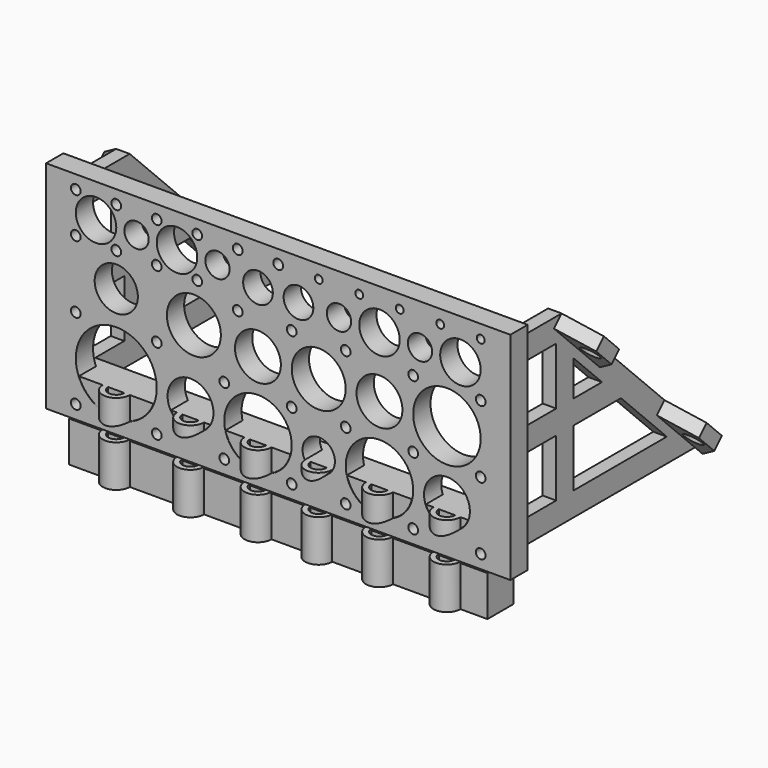
from build123d import *

# Parameters (mm, degrees)
F0_R            = 1.8
F0_R_2          = 1.45
F1_DEPTH        = 8
F2_R            = 8.5
F2_R_2          = 12.5
F2_R_3          = 6
F2_R_4          = 15
F2_R_5          = 8
F2_R_6          = 7.5
F2_R_7          = 4.5
F2_R_8          = 10
F2_R_9          = 5.5
F3_DEPTH        = 8
F4_W            = 5
F4_H            = 5
F5_DEPTH        = 5
F6_W            = 4.8999972641
F6_H            = 4.7999945283
F7_DEPTH        = 5
F11_DEPTH       = 5
F12_DEPTH       = 5
F14_D           = 3.5
F14_CSINK_D     = 7
F14_CSINK_ANGLE = 82
F16_D           = 3.5
F16_CSINK_D     = 7
F16_CSINK_ANGLE = 82
F18_DEPTH       = 12
F20_DEPTH       = 4
F21_DEPTH       = 1
F17_W           = 155
F17_H           = 40
F22_DEPTH       = 12
F17_R           = 1.8
F23_DEPTH       = 25
F24_DEPTH       = 25
F26_DEPTH       = 30
F28_DEPTH       = 25
F25_W           = 13.6818544567
F25_H           = 5
F25_W_2         = 25
F25_W_3         = 22.5
F25_W_4         = 11.7608711123
F29_DEPTH       = 8


with BuildPart() as f1:
    # F0 (on Front) → F1 (new body)
    with BuildSketch(Plane.XZ):
        Polygon((120.2036130428, 95.3458033502), (-39.7963869572, 95.3458033502), (-45.7963869572, 95.3458033502), (-45.7963869572, 15.3458033502), (-39.7963869572, 15.3458033502), (120.2036130428, 15.3458033502), (126.2036130428, 15.3458033502), (126.2036130428, 95.3458033502), align=None)
        with Locations((-34.7963869572, 20.3458033502)):
            Circle(F0_R, mode=Mode.SUBTRACT)
        with Locations((-4.7963869572, 20.3458033502)):
            Circle(F0_R, mode=Mode.SUBTRACT)
        with Locations((20.2036130428, 20.3458033502)):
            Circle(F0_R, mode=Mode.SUBTRACT)
        with Locations((-34.7963869572, 50.3458033502)):
            Circle(F0_R, mode=Mode.SUBTRACT)
        with Locations((-4.7963869572, 50.3458033502)):
            Circle(F0_R, mode=Mode.SUBTRACT)
        with Locations((20.2036130428, 45.3458033502)):
            Circle(F0_R, mode=Mode.SUBTRACT)
        with Locations((45.2036130428, 20.3458033502)):
            Circle(F0_R, mode=Mode.SUBTRACT)
        with Locations((65.2036130428, 20.3458033502)):
            Circle(F0_R, mode=Mode.SUBTRACT)
        with Locations((90.2036130428, 20.3458033502)):
            Circle(F0_R, mode=Mode.SUBTRACT)
        with Locations((115.2036130428, 20.3458033502)):
            Circle(F0_R, mode=Mode.SUBTRACT)
        with Locations((45.2036130428, 45.3458033502)):
            Circle(F0_R, mode=Mode.SUBTRACT)
        with Locations((65.2036130428, 45.3458033502)):
            Circle(F0_R, mode=Mode.SUBTRACT)
        with Locations((90.2036130428, 45.3458033502)):
            Circle(F0_R, mode=Mode.SUBTRACT)
        with Locations((115.2036130428, 45.3458033502)):
            Circle(F0_R, mode=Mode.SUBTRACT)
        with Locations((-34.7963869572, 75.3458033502)):
            Circle(F0_R, mode=Mode.SUBTRACT)
        with Locations((-19.7963869572, 75.3458033502)):
            Circle(F0_R, mode=Mode.SUBTRACT)
        with Locations((-4.7963869572, 75.3458033502)):
            Circle(F0_R, mode=Mode.SUBTRACT)
        with Locations((10.2036130428, 75.3458033502)):
            Circle(F0_R, mode=Mode.SUBTRACT)
        with Locations((25.2036130428, 70.3458033502)):
            Circle(F0_R, mode=Mode.SUBTRACT)
        with Locations((-34.7963869572, 90.3458033502)):
            Circle(F0_R, mode=Mode.SUBTRACT)
        with Locations((-19.7963869572, 90.3458033502)):
            Circle(F0_R, mode=Mode.SUBTRACT)
        with Locations((-4.7963869572, 90.3458033502)):
            Circle(F0_R, mode=Mode.SUBTRACT)
        with Locations((10.2036130428, 90.3458033502)):
            Circle(F0_R, mode=Mode.SUBTRACT)
        with Locations((25.2036130428, 90.3458033502)):
            Circle(F0_R, mode=Mode.SUBTRACT)
        with Locations((45.2036130428, 70.3458033502)):
            Circle(F0_R, mode=Mode.SUBTRACT)
        with Locations((65.2036130428, 70.3458033502)):
            Circle(F0_R, mode=Mode.SUBTRACT)
        with Locations((90.2036130428, 70.3458033502)):
            Circle(F0_R, mode=Mode.SUBTRACT)
        with Locations((115.2036130428, 70.3458033502)):
            Circle(F0_R, mode=Mode.SUBTRACT)
        with Locations((40.2036130428, 90.3458033502)):
            Circle(F0_R, mode=Mode.SUBTRACT)
        with Locations((55.2036130428, 90.3458033502)):
            Circle(F0_R_2, mode=Mode.SUBTRACT)
        with Locations((70.2036130428, 90.3458033502)):
            Circle(F0_R_2, mode=Mode.SUBTRACT)
        with Locations((85.2036130428, 90.3458033502)):
            Circle(F0_R_2, mode=Mode.SUBTRACT)
        with Locations((100.2036130428, 90.3458033502)):
            Circle(F0_R_2, mode=Mode.SUBTRACT)
        with Locations((115.2036130428, 90.3458033502)):
            Circle(F0_R_2, mode=Mode.SUBTRACT)
    extrude(amount=F1_DEPTH)

    # F2 (on face) → F3 (cut)
    with BuildSketch(Plane.XZ.offset(8)):
        with Locations((102.7036130428, 32.8458033502)):
            Circle(F2_R)
        with Locations((77.7036130428, 32.8458033502)):
            Circle(F2_R_2)
        with Locations((55.2036130428, 32.8458033502)):
            Circle(F2_R_3)
        with Locations((32.7036130428, 32.8458033502)):
            Circle(F2_R_2)
        with Locations((7.7036130428, 34.0362795407)):
            Circle(F2_R)
        with Locations((-19.7963869572, 35.3458033502)):
            Circle(F2_R_4)
        with Locations((-19.7963869572, 62.8458033502)):
            Circle(F2_R_5)
        with Locations((-27.2963869572, 82.8458033502)):
            Circle(F2_R_6)
        with Locations((-12.2963869572, 82.8458033502)):
            Circle(F2_R_7)
        with Locations((2.7036130428, 82.8458033502)):
            Circle(F2_R_6)
        with Locations((17.7036130428, 82.8458033502)):
            Circle(F2_R_7)
        with Locations((8.9536130428, 60.3458033502)):
            Circle(F2_R_8)
        with Locations((32.6806940138, 57.8458033502)):
            Circle(F2_R)
        with Locations((55.2036130428, 57.8458033502)):
            Circle(F2_R_8)
        with Locations((77.7036130428, 57.8458033502)):
            Circle(F2_R)
        with Locations((102.7036130428, 57.8458033502)):
            Circle(F2_R_2)
        with Locations((32.7036130428, 80.3458033502)):
            Circle(F2_R_9)
        with Locations((47.7036130428, 80.3458033502)):
            Circle(F2_R_9)
        with Locations((62.7036130428, 80.3458033502)):
            Circle(F2_R_7)
        with Locations((77.7036130428, 80.3458033502)):
            Circle(F2_R_6)
        with Locations((92.7036130428, 80.3458033502)):
            Circle(F2_R_7)
        with Locations((107.7036130428, 80.3458033502)):
            Circle(F2_R_6)
    extrude(amount=-F3_DEPTH, mode=Mode.SUBTRACT)

    # F4 (on face) → F5 (cut)
    with BuildSketch(Plane(origin=(0, 0, 0), x_dir=(-1, 0, 0), z_dir=(0, 1, 0))):
        with Locations((-120.2036130428, 85.3458033502)):
            Rectangle(F4_W, F4_H)
        with Locations((-120.2036130428, 55.3458033502)):
            Rectangle(F4_W, F4_H)
        with Locations((-120.2036130428, 25.3458033502)):
            Rectangle(F4_W, F4_H)
        with Locations((39.7963869572, 25.3458033502)):
            Rectangle(F4_W, F4_H)
        with Locations((39.7963869572, 55.3458033502)):
            Rectangle(F4_W, F4_H)
        with Locations((39.7963869572, 85.3458033502)):
            Rectangle(F4_W, F4_H)
    extrude(amount=-F5_DEPTH, mode=Mode.SUBTRACT)


with BuildPart() as f7:
    # F6 (on face) → F7 (new body)
    with BuildSketch(Plane.YZ.offset(117.7036130428)):
        Polygon((0.0999999975, 87.7458006144), (0, 87.7458006144), (0, 82.9458060861), (0.0999999975, 82.9458060861), (0.0999999975, 80.9458060861), (5.0999999975, 80.9458060861), (17.5862857401, 80.9458060861), (17.5862857401, 59.7458031476), (5.0999999975, 59.7458031476), (0.0999999975, 59.7458031476), (0.0999999975, 57.7458031476), (0, 57.7458031476), (-4.8999997973, 57.7458031476), (-4.8999997973, 52.9458035529), (0, 52.9458035529), (0.0999999975, 52.9458035529), (0.0999999975, 50.9458035529), (5.0999999975, 50.9458035529), (17.5862857401, 50.9458035529), (17.5862857401, 29.7458038181), (5.0999999975, 29.7458038181), (0.0999999975, 29.7458038181), (0.0999999975, 27.7458038181), (0, 27.7458038181), (-4.9000004679, 27.7458038181), (-4.9000004679, 22.9458028823), (0, 22.9458028823), (0.0999999975, 22.9458028823), (0.0999999975, 20.9458028823), (5.0999999975, 20.9458028823), (88.8999977295, 20.9458028823), (20.0999999975, 89.7458006144), (5.0999999975, 89.7458006144), (0.0999999975, 89.7458006144), align=None)
        Polygon((25.5862857401, 50.9458035529), (47.5862882733, 50.9458035529), (68.7862880081, 29.7458038181), (25.5862857401, 29.7458038181), align=None, mode=Mode.SUBTRACT)
        Polygon((25.5862857401, 59.7458031476), (25.5862857401, 72.9458060861), (38.7862886786, 59.7458031476), align=None, mode=Mode.SUBTRACT)
        with Locations((-2.4499986321, 85.3458033502)):
            Rectangle(F6_W, F6_H)
    extrude(amount=F7_DEPTH)


with BuildPart() as f8_1:
    # F8: copy of F7
    add(f7.part.moved(Location((-160, 0, 0))))

    # F10 (on face) → F12 (join)
    with BuildSketch(Plane(origin=(0, 54.9229003059, 54.9229003059), x_dir=(-1, 0, 0), z_dir=(0, 0.7071067812, 0.7071067812))):
        Polygon((42.2963869572, 49.2470178974), (42.2963869572, 19.2470178974), (52.2963869572, 29.2470178974), (52.2963869572, 39.2470178974), align=None)
        Polygon((42.2963869572, -18.0508719865), (42.2963869572, -48.0508719865), (52.2963869572, -38.0508719865), (52.2963869572, -28.0508719865), align=None)
    extrude(amount=-F12_DEPTH)

    # F14 (through all)
    with Locations(Plane(origin=(0, 51.3873664, 51.3873664), x_dir=(1, 0, 0), z_dir=(0, -0.7071067812, -0.7071067812))):
        with Locations((-47.2963869572, 34.2470178974), (-47.2963869572, -33.0508719865)):
            CounterSinkHole(F14_D / 2, F14_CSINK_D / 2, counter_sink_angle=F14_CSINK_ANGLE)


with BuildPart() as f7_1:
    add(f7.part)

    # F9 (on face) → F11 (join)
    with BuildSketch(Plane(origin=(0, 54.9229003059, 54.9229003059), x_dir=(-1, 0, 0), z_dir=(0, 0.7071067812, 0.7071067812))):
        Polygon((-122.7036130428, 19.2470178974), (-122.7036130428, 49.2470178974), (-132.7036130428, 39.2470178974), (-132.7036130428, 29.2470178974), align=None)
        Polygon((-122.7036130428, -48.0508719865), (-122.7036130428, -18.0508719865), (-132.7036130428, -28.0508719865), (-132.7036130428, -38.0508719865), align=None)
    extrude(amount=-F11_DEPTH)

    # F16 (through all)
    with Locations(Plane(origin=(0, 51.3873664, 51.3873664), x_dir=(1, 0, 0), z_dir=(0, -0.7071067812, -0.7071067812))):
        with Locations((127.7036130428, 34.2470178974), (127.7036130428, -33.0508719865)):
            CounterSinkHole(F16_D / 2, F16_CSINK_D / 2, counter_sink_angle=F16_CSINK_ANGLE)


with BuildPart() as f18:
    # F17 (on face) → F18 (new body)
    with BuildSketch(Plane.XZ.offset(8)):
        with BuildLine():
            Line((-5.9486424639, 29.8458033502), (-33.6441314504, 29.8458033502))
            ThreePointArc((-33.6441314504, 29.8458033502), (-19.7963869572, 20.4458024257), (-5.9486424639, 29.8458033502))
        make_face()
    extrude(amount=-F18_DEPTH)



with BuildPart() as f18b:
    # F17 (on face) → F18, piece 2 (new body)
    with BuildSketch(Plane.XZ.offset(8)):
        with BuildLine():
            Line((14.9837176064, 29.8458033502), (0.4235084793, 29.8458033502))
            ThreePointArc((0.4235084793, 29.8458033502), (7.7036130428, 25.6362787574), (14.9837176064, 29.8458033502))
        make_face()
    extrude(amount=-F18_DEPTH)


with BuildPart() as f18c:
    # F17 (on face) → F18, piece 3 (new body)
    with BuildSketch(Plane.XZ.offset(8)):
        with BuildLine():
            Line((44.735236756, 29.8458033502), (20.6719893297, 29.8458033502))
            ThreePointArc((20.6719893297, 29.8458033502), (32.7036130428, 20.4458045932), (44.735236756, 29.8458033502))
        make_face()
    extrude(amount=-F18_DEPTH)


with BuildPart() as f18d:
    # F17 (on face) → F18, piece 4 (new body)
    with BuildSketch(Plane.XZ.offset(8)):
        with BuildLine():
            ThreePointArc((50.1232573727, 29.8458033502), (55.2036130428, 26.9458021862), (60.2839687129, 29.8458033502))
            Line((60.2839687129, 29.8458033502), (50.1232573727, 29.8458033502))
        make_face()
    extrude(amount=-F18_DEPTH)


with BuildPart() as f18e:
    # F17 (on face) → F18, piece 5 (new body)
    with BuildSketch(Plane.XZ.offset(8)):
        with BuildLine():
            ThreePointArc((65.6719880487, 29.8458033502), (77.7036130428, 20.4458033502), (89.735238037, 29.8458033502))
            Line((89.735238037, 29.8458033502), (65.6719880487, 29.8458033502))
        make_face()
    extrude(amount=-F18_DEPTH)


with BuildPart() as f18f:
    # F17 (on face) → F18, piece 6 (new body)
    with BuildSketch(Plane.XZ.offset(8)):
        with BuildLine():
            ThreePointArc((94.857596597, 29.8458033502), (102.7036130428, 24.4458048937), (110.5496294887, 29.8458033502))
            Line((110.5496294887, 29.8458033502), (94.857596597, 29.8458033502))
        make_face()
    extrude(amount=-F18_DEPTH)


with BuildPart() as f18_1:
    add(f18.part)

    add(f18b.part)  # F20 merges F18b

    add(f18c.part)  # F20 merges F18c

    add(f18d.part)  # F20 merges F18d

    add(f18e.part)  # F20 merges F18e

    add(f18f.part)  # F20 merges F18f
    # F19 (on face) → F20 (join)
    with BuildSketch(Plane(origin=(0, 0, 0), x_dir=(-1, 0, 0), z_dir=(0, 1, 0))):
        Polygon((37.2963869572, 29.8458033502), (33.6441314504, 29.8458033502), (5.9486424639, 29.8458033502), (-117.7036130428, 29.8458033502), (-117.7036130428, 20.9458028823), (-117.7036130428, 15.3458033502), (37.2963869572, 15.3458033502), (37.2963869572, 20.9458028823), align=None)
    extrude(amount=F20_DEPTH)

    # F21 (add): a face of the model
    f21_faces = [f18_1.faces().sort_by_distance(p)[0] for p in [
        (40.2036130428, 2, 15.3458033502),
    ]]
    extrude(f21_faces, amount=F21_DEPTH)

    # F17 (on face) → F22 (join)
    with BuildSketch(Plane.XZ.offset(8)):
        with Locations((40.2036130428, -5.1541966498)):
            Rectangle(F17_W, F17_H)
    extrude(amount=-F22_DEPTH)

    # F17 (on face) → F23 (cut)
    with BuildSketch(Plane.XZ.offset(8)):
        with Locations((-34.7963869572, 20.3458033502)):
            Circle(F17_R)
        with Locations((-4.7963869572, 20.3458033502)):
            Circle(F17_R)
        with Locations((20.2036130428, 20.3458033502)):
            Circle(F17_R)
        with Locations((45.2036130428, 20.3458033502)):
            Circle(F17_R)
        with Locations((65.2036130428, 20.3458033502)):
            Circle(F17_R)
        with Locations((90.2036130428, 20.3458033502)):
            Circle(F17_R)
        with Locations((115.2036130428, 20.3458033502)):
            Circle(F17_R)
    extrude(amount=-F23_DEPTH, mode=Mode.SUBTRACT)

    # F24 (cut): a face of the model
    f24_faces = [f18_1.faces().sort_by_distance(p)[0] for p in [
        (40.2036130428, -2, -25.1541966498),
    ]]
    extrude(f24_faces, amount=-F24_DEPTH, mode=Mode.SUBTRACT)

    # F25 (on face) → F26 (join)
    with BuildSketch(Plane(origin=(0, 0, -0.1541966498), x_dir=(1, 0, 0), z_dir=(0, 0, -1))):
        with BuildLine():
            ThreePointArc((-14.7963869572, 8), (-19.7963869572, 13), (-24.7963869572, 8))
            Line((-24.7963869572, 8), (-22.7963869572, 8))
            ThreePointArc((-22.7963869572, 8), (-19.7963869572, 11), (-16.7963869572, 8))
            Line((-16.7963869572, 8), (-14.7963869572, 8))
        make_face()
        with BuildLine():
            ThreePointArc((12.7036130428, 8), (7.7036130428, 13), (2.7036130428, 8))
            Line((2.7036130428, 8), (4.7036130428, 8))
            ThreePointArc((4.7036130428, 8), (7.7036130428, 11), (10.7036130428, 8))
            Line((10.7036130428, 8), (12.7036130428, 8))
        make_face()
        with BuildLine():
            ThreePointArc((37.7036130428, 8), (32.7036130428, 13), (27.7036130428, 8))
            Line((27.7036130428, 8), (29.7036130428, 8))
            ThreePointArc((29.7036130428, 8), (32.7036130428, 11), (35.7036130428, 8))
            Line((35.7036130428, 8), (37.7036130428, 8))
        make_face()
        with BuildLine():
            Line((58.2036130428, 8), (60.2036130428, 8))
            ThreePointArc((60.2036130428, 8), (55.2036130428, 13), (50.2036130428, 8))
            Line((50.2036130428, 8), (52.2036130428, 8))
            ThreePointArc((52.2036130428, 8), (55.2036130428, 11), (58.2036130428, 8))
        make_face()
        with BuildLine():
            Line((80.7036130428, 8), (82.7036130428, 8))
            ThreePointArc((82.7036130428, 8), (77.7036130428, 13), (72.7036130428, 8))
            Line((72.7036130428, 8), (74.7036130428, 8))
            ThreePointArc((74.7036130428, 8), (77.7036130428, 11), (80.7036130428, 8))
        make_face()
        with BuildLine():
            Line((105.7036130428, 8), (107.7036130428, 8))
            ThreePointArc((107.7036130428, 8), (102.7036130428, 13), (97.7036130428, 8))
            Line((97.7036130428, 8), (99.7036130428, 8))
            ThreePointArc((99.7036130428, 8), (102.7036130428, 11), (105.7036130428, 8))
        make_face()
    extrude(amount=-F26_DEPTH)

    # F27 (on face) → F28 (cut)
    with BuildSketch(Plane.XZ.offset(8)):
        with BuildLine():
            Line((-24.7963869572, 18.0777903203), (-24.7963869572, 15.3458033502))
            Line((-24.7963869572, 15.3458033502), (-14.7963869572, 15.3458033502))
            Line((-14.7963869572, 15.3458033502), (-14.7963869572, 18.0777903203))
            Line((-14.7963869572, 18.0777903203), (-14.7963869572, 21.2036677265))
            ThreePointArc((-14.7963869572, 21.2036677265), (-19.7963869572, 20.3458033502), (-24.7963869572, 21.2036677265))
            Line((-24.7963869572, 21.2036677265), (-24.7963869572, 18.0777903203))
        make_face()
        with BuildLine():
            Line((2.7036130428, 27.1624159983), (2.7036130428, 15.3458033502))
            Line((2.7036130428, 15.3458033502), (12.7036130428, 15.3458033502))
            Line((12.7036130428, 15.3458033502), (12.7036130428, 27.1624159983))
            ThreePointArc((12.7036130428, 27.1624159983), (7.7036130428, 25.5362795407), (2.7036130428, 27.1624159983))
        make_face()
        with BuildLine():
            Line((27.7036130428, 15.3458033502), (37.7036130428, 15.3458033502))
            Line((37.7036130428, 15.3458033502), (37.7036130428, 21.3893641128))
            ThreePointArc((37.7036130428, 21.3893641128), (32.7036130428, 20.3458033502), (27.7036130428, 21.3893641128))
            Line((27.7036130428, 21.3893641128), (27.7036130428, 15.3458033502))
        make_face()
        with BuildLine():
            Line((72.7036130428, 15.3458033502), (82.7036130428, 15.3458033502))
            Line((82.7036130428, 15.3458033502), (82.7036130428, 21.3893641128))
            ThreePointArc((82.7036130428, 21.3893641128), (77.7036130428, 20.3458033502), (72.7036130428, 21.3893641128))
            Line((72.7036130428, 21.3893641128), (72.7036130428, 15.3458033502))
        make_face()
        with BuildLine():
            Line((97.7036130428, 15.3458033502), (107.7036130428, 15.3458033502))
            Line((107.7036130428, 15.3458033502), (107.7036130428, 25.9719398078))
            ThreePointArc((107.7036130428, 25.9719398078), (102.7036130428, 24.3458033502), (97.7036130428, 25.9719398078))
            Line((97.7036130428, 25.9719398078), (97.7036130428, 15.3458033502))
        make_face()
        with BuildLine():
            Line((50.2036130428, 15.3458033502), (60.2036130428, 15.3458033502))
            Line((60.2036130428, 15.3458033502), (60.2036130428, 29.5291785599))
            ThreePointArc((60.2036130428, 29.5291785599), (55.2036130428, 26.8458033502), (50.2036130428, 29.5291785599))
            Line((50.2036130428, 29.5291785599), (50.2036130428, 15.3458033502))
        make_face()
    extrude(amount=F28_DEPTH, mode=Mode.SUBTRACT)

    # F25 (on face) → F29 (cut)
    with BuildSketch(Plane(origin=(0, 0, -0.1541966498), x_dir=(1, 0, 0), z_dir=(0, 0, -1))):
        with Locations((-26.6373141855, 2)):
            Rectangle(F25_W, F25_H)
        with Locations((20.2036130428, 2)):
            Rectangle(F25_W_2, F25_H)
        with Locations((66.4536130428, 2)):
            Rectangle(F25_W_3, F25_H)
        with Locations((108.584048599, 2)):
            Rectangle(F25_W_4, F25_H)
    extrude(amount=-F29_DEPTH, mode=Mode.SUBTRACT)


solid = Compound([f1.part, f8_1.part, f7_1.part, f18_1.part])
